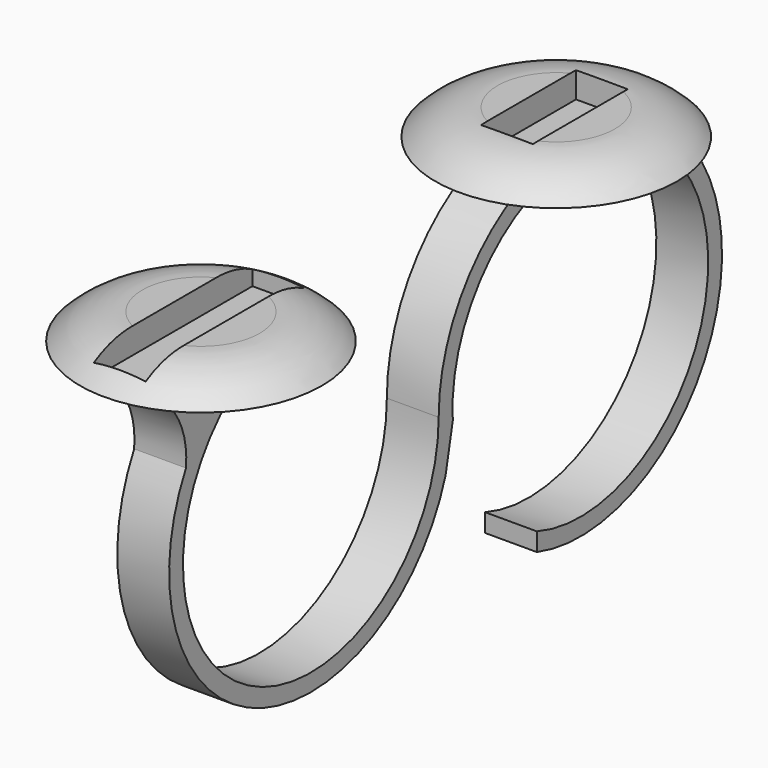
from build123d import *

# Parameters (mm, degrees)
F1_DEPTH = 3
F2_R     = 7
F2_W     = 3
F2_H     = 11.476257816
F3_DEPTH = 1.5
F5_R     = 7
F5_W     = 3
F5_H     = 6.8703614243
F6_DEPTH = 1.5


# Not quite as in the source:
# - a fillet or chamfer that OpenCascade refuses, or shapes differently, is made with other operations: its cross-section is extruded or revolved along the edge and cut away or added


with BuildPart() as f1:
    # F0 (on Right) → F1 (new body)
    with BuildSketch(Plane.YZ):
        with BuildLine():
            ThreePointArc((-9.23076647, -0.5961965923), (7.3973798388, 5.5534918313), (-3.1487550555, -8.697576766))
            Line((-3.1487550555, -8.697576766), (-3.1487550555, -9.7543755105))
            ThreePointArc((-3.1487550555, -9.7543755105), (9.7068577817, -3.2923262302), (3.4351807121, 9.6572270075))
            Line((3.4351807121, 9.6572270075), (-3.4351807121, 9.6572270075))
            ThreePointArc((-3.4351807121, 9.6572270075), (-8.3747567815, 5.9098180048), (-10.25, 0))
            ThreePointArc((-10.25, 0), (-25.8708649083, -6.7063089937), (-19.9742335826, 9.2378353801))
            Line((-19.9742335826, 9.2378353801), (-19.9742335826, 9.6572270075))
            Line((-19.9742335826, 9.6572270075), (-22.9351807121, 9.6572270075))
            Line((-22.9351807121, 9.6572270075), (-31.4504913986, 9.6572270075))
            ThreePointArc((-31.4504913986, 9.6572270075), (-29.1894054573, 7.7380849014), (-28.5320347977, 4.8461167354))
            ThreePointArc((-28.5320347977, 4.8461167354), (-23.5202566717, -9.4286815777), (-9.75, -3.1622776602))
            Line((-9.75, -3.1622776602), (-9.23076647, -0.5961965923))
        make_face()
    extrude(amount=F1_DEPTH)


with BuildPart() as f3:
    # F2 (on face) → F3 (new body)
    with BuildSketch(Plane.XY.offset(9.6572270075)):
        with Locations((1.5416375827, -25.6245899945)):
            Circle(F2_R)
        with Locations((1.5, -25.7123624906)):
            Rectangle(F2_W, F2_H, mode=Mode.SUBTRACT)
    extrude(amount=F3_DEPTH)

    # F4: fillet of radius 5.08 on 1 edges, made by hand

    # F4_s1 → F4_t2 (revolve, cut)
    with BuildSketch(Plane.XZ.offset(25.6245899945)):
        with BuildLine():
            ThreePointArc((8.5416375827, 9.6572270075), (6.8893954541, 10.7672589904), (4.9374733245, 11.1572270075))
            Line((4.9374733245, 11.1572270075), (8.5416375827, 11.1572270075))
            Line((8.5416375827, 11.1572270075), (8.5416375827, 9.6572270075))
        make_face()
    revolve(axis=Axis((1.5416375827, -25.6245899945, 11.1572270075), (0, 0, 1)), mode=Mode.SUBTRACT)


with BuildPart() as f6:
    # F5 (on face) → F6 (new body)
    with BuildSketch(Plane.XY.offset(9.6572270075)):
        with Locations((1.581404591, 0.0261381756)):
            Circle(F5_R)
        with Locations((1.5, 0)):
            Rectangle(F5_W, F5_H, mode=Mode.SUBTRACT)
    extrude(amount=F6_DEPTH)

    # F7: fillet of radius 5.08 on 1 edges, made by hand

    # F7_s1 → F7_t2 (revolve, cut)
    with BuildSketch(Plane.XZ.offset(-0.0261381756)):
        with BuildLine():
            ThreePointArc((8.581404591, 9.6572270075), (6.9291624624, 10.7672589904), (4.9772403328, 11.1572270075))
            Line((4.9772403328, 11.1572270075), (8.581404591, 11.1572270075))
            Line((8.581404591, 11.1572270075), (8.581404591, 9.6572270075))
        make_face()
    revolve(axis=Axis((1.581404591, 0.0261381756, 11.1572270075), (0, 0, 1)), mode=Mode.SUBTRACT)


solid = Compound([f1.part, f3.part, f6.part])
